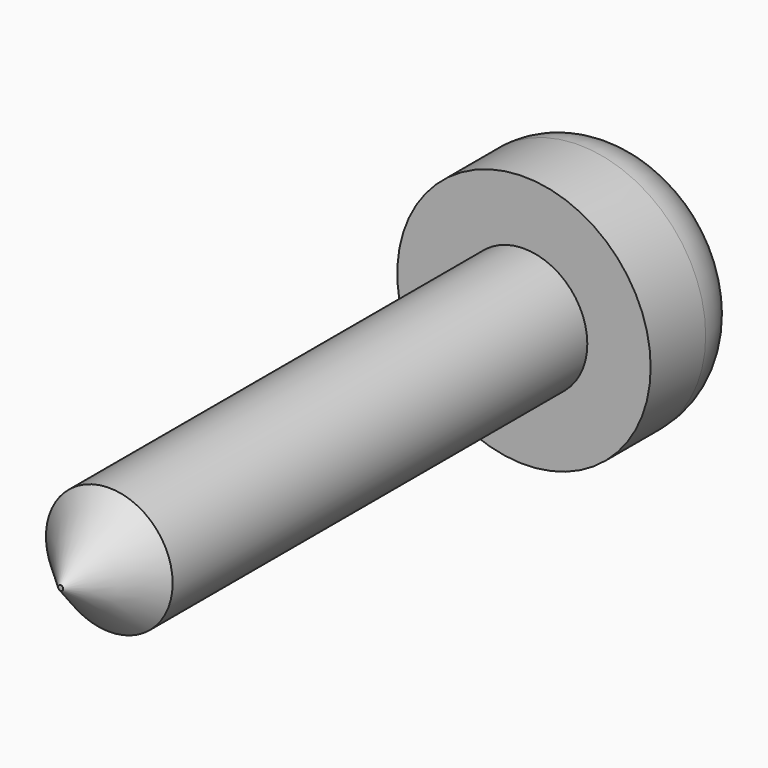
from build123d import *

# Parameters (mm, degrees)
F0_R     = 2.778125
F1_DEPTH = 1.3890625
F2_R     = 1.3890625
F3_DEPTH = 12.7
F4_W     = 0.79375
F4_H     = 3.175
F6_DEPTH = 2.38125
F5_W     = 3.175
F5_H     = 0.79375
F7_DEPTH = 2.38125
F8_R     = 0.127
F10_SIZE = 1.3335


# Not quite as in the source:
# - a fillet or chamfer that OpenCascade refuses, or shapes differently, is made with other operations: its cross-section is extruded or revolved along the edge and cut away or added


with BuildPart() as f1:
    # F0 (on Front) → F1 (new body, symmetric)
    with BuildSketch(Plane.XZ):
        Circle(F0_R)
    extrude(amount=F1_DEPTH, both=True)

    # F2 (on face) → F3 (join)
    with BuildSketch(Plane.XZ.offset(1.3890625)):
        Circle(F2_R)
    extrude(amount=F3_DEPTH)

    # F4 (on face) → F6 (cut)
    with BuildSketch(Plane(origin=(0, 1.3890625, 0), x_dir=(-1, 0, 0), z_dir=(0, 1, 0))):
        Rectangle(F4_W, F4_H)
    extrude(amount=-F6_DEPTH, mode=Mode.SUBTRACT)

    # F5 (on face) → F7 (cut)
    with BuildSketch(Plane(origin=(0, 1.3890625, 0), x_dir=(-1, 0, 0), z_dir=(0, 1, 0))):
        Rectangle(F5_W, F5_H)
    extrude(amount=-F7_DEPTH, mode=Mode.SUBTRACT)

    # F8
    f8_edges = [f1.edges().sort_by_distance(p)[0] for p in [
        (0.396875, 0.198438, 0.396875),
        (-0.396875, 0.198438, 0.396875),
        (-0.396875, 0.198438, -0.396875),
        (0.396875, 0.198438, -0.396875),
    ]]
    fillet(f8_edges, radius=F8_R)

    # F9: fillet of radius 1.27 on 1 edges, made by hand

    # F9_s1 → F9_t2 (revolve, cut)
    with BuildSketch(Plane.XY):
        with BuildLine():
            ThreePointArc((1.508125, 1.3890625), (2.4061506121, 1.0170881121), (2.778125, 0.1190625))
            Line((2.778125, 0.1190625), (2.778125, 1.3890625))
            Line((2.778125, 1.3890625), (1.508125, 1.3890625))
        make_face()
    revolve(axis=Axis((0, 1.3890625, 0), (0, -1, 0)), mode=Mode.SUBTRACT)

    # F10
    f10_edges = [f1.edges().sort_by_distance(p)[0] for p in [
        (-1.389062, -14.089062, 0),
    ]]
    chamfer(f10_edges, length=F10_SIZE)


solid = f1.part
